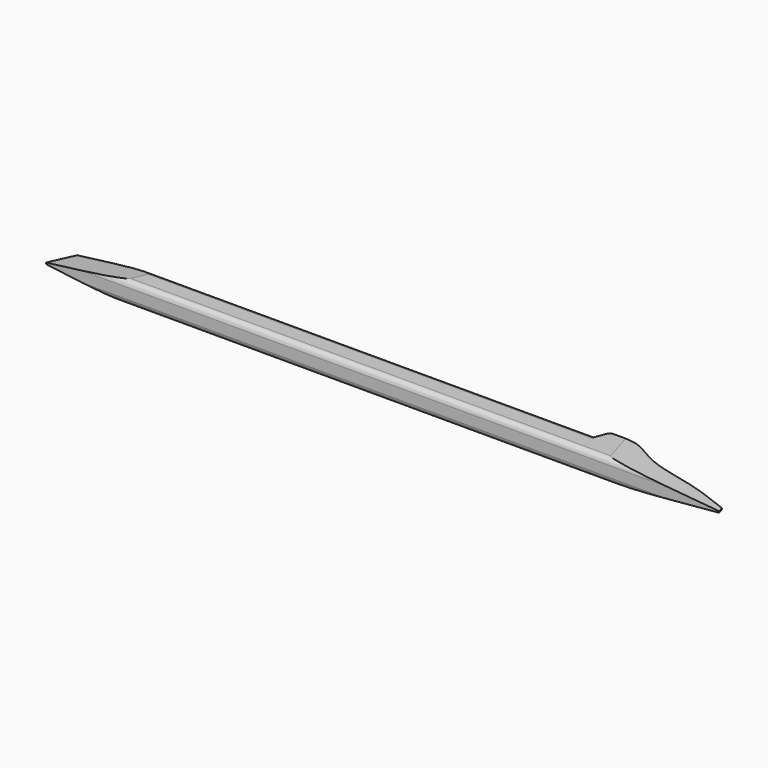
from build123d import *

# Parameters (mm, degrees)
F1_DEPTH     = 6
F2_T1_DEPTH  = 157.6354832979
F3_T1_DEPTH  = 180.911939444
F3_T3_DEPTH  = 11.1833176621
F3_T8_DEPTH  = 154.2537676368
F3_T13_DEPTH = 154.2537676368
F4_T1_DEPTH  = 108.3530023153


# Not quite as in the source:
# - a fillet or chamfer that OpenCascade refuses, or shapes differently, is made with other operations: its cross-section is extruded or revolved along the edge and cut away or added


with BuildPart() as f1:
    # F0 (on Top) → F1 (new body)
    with BuildSketch(Plane.XY):
        Polygon((38.1666665349, 7), (-81.8333334651, 7), (-81.8333334651, 0), (38.5162681341, 0), align=None)
        with BuildLine():
            Line((39.3004275709, 10), (38.1666665349, 7))
            Line((38.1666665349, 7), (38.5162681341, 0))
            Line((38.5162681341, 0), (46.4909672737, 0))
            Line((46.4909672737, 0), (77.9909640551, 0))
            Line((77.9909640551, 0), (77.5119066238, 1.5898427228))
            add(Edge.make_bspline(
                [(46.4909672737, 10), (49.5646846807, 9.1582136368), (54.0969093449, 5.5068681922), (67.4802237728, 4.9316783562), (74.0574866156, 2.5085939236), (77.5119066238, 1.5898427228)],
                knots=[0, 0, 0, 0, 0.3024831153, 0.6658844955, 1, 1, 1, 1], degree=3))
            Line((46.4909672737, 10), (39.3004275709, 10))
        make_face()
        Polygon((-81.8333334651, 0), (-81.8333334651, 7), (-108.5871011019, 7), (-111.7533296347, 0), align=None)
    extrude(amount=F1_DEPTH)

    # F2: chamfer of 30 x 2.8 on 2 edges, made by hand

    # F2_s2 → F2_t1 (cut)
    with BuildSketch(Plane(origin=(28.992055027, -96.2156198783, 0), x_dir=(0, 0, 1), z_dir=(-0.2885105142, 0.9574767272, 0))):
        Polygon((3.2, 74.6745330178), (6, 44.6745330178), (6, 74.6745330178), align=None)
        Polygon((2.8, 74.6745330178), (0, 44.6745330178), (0, 74.6745330178), align=None)
    extrude(amount=F2_T1_DEPTH, mode=Mode.SUBTRACT)

    # F3: fillet of radius 1.5 on 5 edges, made by hand

    # F3_s2 → F3_t1 (cut)
    with BuildSketch(Plane.YZ.offset(-115.5033296347)):
        with BuildLine():
            ThreePointArc((1.5, 6), (0.4393398282, 5.5606601718), (0, 4.5))
            Line((0, 4.5), (0, 6))
            Line((0, 6), (1.5, 6))
        make_face()
        with BuildLine():
            ThreePointArc((1.5, 0), (0.4393398282, 0.4393398282), (0, 1.5))
            Line((0, 1.5), (0, 0))
            Line((0, 0), (1.5, 0))
        make_face()
    extrude(amount=F3_T1_DEPTH, mode=Mode.SUBTRACT)

    # F3_s4 → F3_t3 (cut)
    with BuildSketch(Plane.XY.offset(-2.591658831)):
        with BuildLine():
            ThreePointArc((38.9339491071, 9.0302759078), (39.4842763115, 9.7339801177), (40.3370911034, 10))
            Line((40.3370911034, 10), (39.3004275709, 10))
            Line((39.3004275709, 10), (38.9339491071, 9.0302759078))
        make_face()
    extrude(amount=F3_T3_DEPTH, mode=Mode.SUBTRACT)


with BuildPart() as f3_tool6:
    # F3_s7 → F3_t8 (new body)
    with BuildSketch(Plane.YZ.offset(41.9166665349)):
        with BuildLine():
            ThreePointArc((7, 4.5), (6.5606601718, 5.5606601718), (5.5, 6))
            Line((5.5, 6), (7, 6))
            Line((7, 6), (7, 4.5))
        make_face()
    extrude(amount=-F3_T8_DEPTH)

    split(bisect_by=Plane(origin=(31.0819782613, -11.7465119587, 0), x_dir=(0, 0, 1), z_dir=(-0.9354279975, 0.3535172719, 0)), keep=Keep.TOP)


with BuildPart() as f1_1:
    add(f1.part)

    # F3_t5: cut F3_tool6
    add(f3_tool6.part, mode=Mode.SUBTRACT)


with BuildPart() as f3_tool11:
    # F3_s12 → F3_t13 (new body)
    with BuildSketch(Plane.YZ.offset(41.9166665349)):
        with BuildLine():
            ThreePointArc((7, 1.5), (6.5606601718, 0.4393398282), (5.5, 0))
            Line((5.5, 0), (7, 0))
            Line((7, 0), (7, 1.5))
        make_face()
    extrude(amount=-F3_T13_DEPTH)

    split(bisect_by=Plane(origin=(31.0819782613, -11.7465119587, 0), x_dir=(0, 0, 1), z_dir=(-0.9354279975, 0.3535172719, 0)), keep=Keep.TOP)


with BuildPart() as f1_2:
    add(f1_1.part)

    # F3_t10: cut F3_tool11
    add(f3_tool11.part, mode=Mode.SUBTRACT)

    # F4: chamfer of 20 x 2.8 on 2 edges, made by hand

    # F4_s2 → F4_t1 (cut)
    with BuildSketch(Plane(origin=(4.9298048814, 10.8989713826, 0), x_dir=(0, 0, 1), z_dir=(-0.4121205293, -0.9111293373, 0))):
        Polygon((6, 81.8217371748), (3.2, 101.8217371748), (6, 101.8217371748), align=None)
        Polygon((0, 81.8217371748), (2.8, 101.8217371748), (0, 101.8217371748), align=None)
    extrude(amount=F4_T1_DEPTH, mode=Mode.SUBTRACT)


solid = f1_2.part
